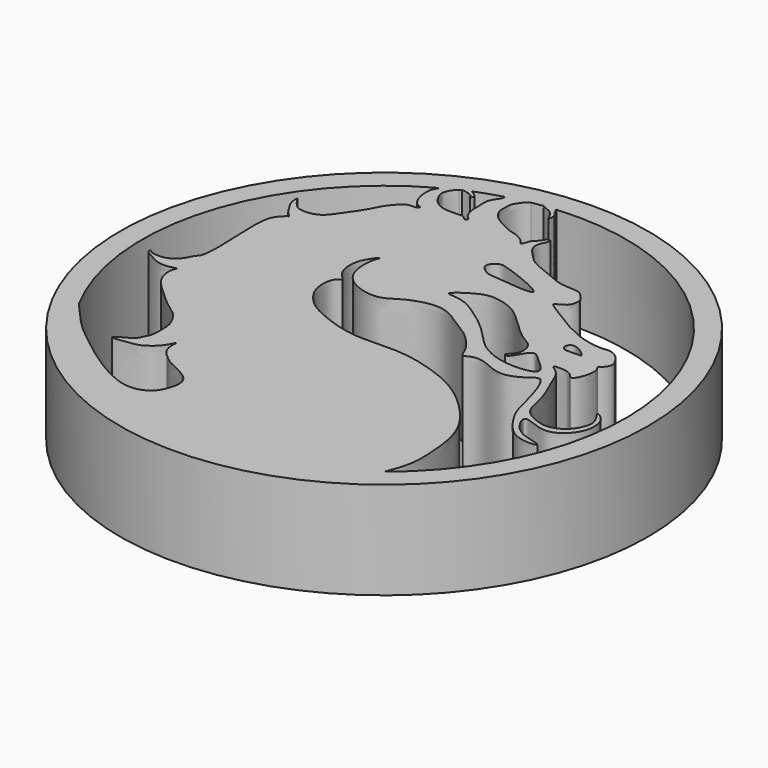
from build123d import *

# Parameters (mm, degrees)
F0_R     = 31.6990102439
F1_DEPTH = 11.7


with BuildPart() as f1:
    # F0 (on Top) → F1 (new body)
    with BuildSketch(Plane.XY):
        Circle(F0_R)
        with BuildLine():
            add(Edge.make_bspline(
                [(-25.4924991119, -13.953342914), (-24.5205169338, -15.0949653302), (-22.7712795464, -17.0908646211), (-20.9172889954, -18.6531879557), (-18.2968648266, -20.6691769997), (-16.0576388328, -22.2866539049), (-12.4835639639, -24.2367282269), (-10.1908173872, -24.1443080261), (-8.8516569375, -23.3219450661), (-8.2884059782, -22.1940801251), (-7.925939069, -20.9577066664), (-8.1157075896, -19.5625424569), (-9.9910246166, -18.4916373157), (-11.2641391672, -17.9900335901), (-12.2342182318, -17.2485160801), (-13.2039862501, -16.3164485705), (-13.4759813903, -15.2533092584), (-13.3229134314, -14.1868992615), (-13.7130330942, -15.0105365297), (-14.1891719411, -15.812497329), (-15.0326748195, -16.5008887465), (-15.8548336143, -17.0523376609), (-17.2619658719, -17.1641585773), (-17.9396597588, -17.310965029), (-19.0370830117, -17.4300508562), (-18.635512969, -16.9608620996), (-17.8651450299, -16.6343730103), (-17.1300961664, -16.1576111235), (-16.70189117, -15.7281851081), (-16.544862205, -15.1135475957), (-16.1178720626, -14.6375624469), (-16.1170114575, -12.1417295665), (-16.5073688058, -11.2488630843), (-17.1586601796, -10.0698478487), (-18.2395336648, -9.334157054), (-19.4351823142, -8.4220615411), (-20.9023358044, -7.0480236886), (-22.051850097, -6.0235129872), (-22.9560730456, -4.7224379727), (-23.1145722043, -3.1268944114), (-22.6189057646, -2.4703301229), (-23.4564204373, -2.768219693), (-24.2140705088, -2.8630415189), (-25.2546086687, -2.6946099421), (-26.1534811662, -2.0869842562), (-27.2257353007, -1.6017665898), (-27.0135812832, -1.1960557968), (-26.7692309783, -1.4218595095), (-26.6222190112, -1.5577130252)],
                knots=[0, 0, 0, 0, 0.0398660387, 0.0704586732, 0.1051574303, 0.1385907296, 0.1775557103, 0.2064699431, 0.2298732252, 0.2514273797, 0.2733952533, 0.2953631269, 0.3232816075, 0.3464860594, 0.3678132978, 0.3901099659, 0.4113282877, 0.427165272, 0.4411293294, 0.461100555, 0.4811676125, 0.5007036306, 0.5232544455, 0.5411884608, 0.5585369833, 0.5695176296, 0.5880729408, 0.6064731354, 0.6214715959, 0.6362150192, 0.6516876832, 0.6817388171, 0.7019175478, 0.7237519879, 0.7459225483, 0.7700142909, 0.7976991764, 0.8220278718, 0.8465425239, 0.8711245294, 0.8844079913, 0.8992487966, 0.9173023826, 0.9367348376, 0.95807413, 0.9778676473, 0.9866834549, 1, 1, 1, 1], degree=3))
            ThreePointArc((-25.4924991119, -13.953342914), (-27.8223142289, 8.2534102291), (-13.7385207838, 25.5801146426))
            add(Edge.make_bspline(
                [(-24.8989164829, -1.5577130252), (-24.6682612127, -1.4467950062), (-24.182278602, -1.2130946081), (-23.5284769239, -0.5252534093), (-23.1348921367, 0.5509903957), (-22.248480301, 0.9536932892), (-22.6348383075, 7.7223592702), (-22.6502976613, 8.636841393), (-22.5815628754, 10.3935904447), (-22.1575913528, 11.4418886666), (-21.3881202113, 12.1606956989), (-21.1235642698, 12.2680174337), (-21.8063168168, 12.7530703595), (-22.1396372934, 13.415098283), (-22.6935277447, 14.1650088888), (-22.8842543668, 14.8759577126), (-22.9465718409, 15.8082146545), (-22.559642771, 15.0793561333), (-22.1324554976, 14.5388286717), (-21.6979561921, 14.0895012776), (-20.9015910939, 13.8854920097), (-19.825223354, 13.9570235717), (-18.8458738409, 14.3881421588), (-18.071126134, 15.4033010207), (-17.2606622947, 16.5246614142), (-16.1601092221, 18.2494885912), (-15.6607329457, 19.3859623739), (-14.847256475, 20.4158034631), (-14.0235241732, 21.1839127113), (-12.9636520335, 21.0055073847), (-12.6225680971, 21.4021121154), (-13.3643600704, 21.5526818883), (-13.9976499307, 22.4695994422), (-14.3470936559, 24.0526739486), (-14.1182749531, 24.987729418), (-13.8062536012, 25.4899631194), (-13.7385207838, 25.5801146426)],
                knots=[0, 0, 0, 0, 0.0256023524, 0.0539148324, 0.0835052959, 0.1101156606, 0.1835979514, 0.2157474491, 0.2521308262, 0.2841448995, 0.3131193533, 0.3242716257, 0.3479291799, 0.3742971001, 0.4016912477, 0.4283317743, 0.4503249132, 0.4705478815, 0.4962303529, 0.5185566477, 0.5442746968, 0.5743387515, 0.603924567, 0.635986405, 0.6708293895, 0.7121609059, 0.7449046934, 0.77779553, 0.8080446572, 0.8370290557, 0.8523168513, 0.8735942078, 0.9042708295, 0.9410102592, 0.9713895558, 0.988723741, 0.988723741, 0.988723741, 0.988723741], degree=3))
            ThreePointArc((-24.8989164829, -1.5577130252), (-25.7605677471, -1.6476774835), (-26.6222190112, -1.5577130252))
        make_face(mode=Mode.SUBTRACT)
        with BuildLine():
            add(Edge.make_bspline(
                [(-10.9293263316, 26.9279244537), (-10.7761460856, 27.1829858205), (-8.4632358732, 28.0968939132), (-7.96494233, 27.9485774795)],
                knots=[0.9212322924, 0.9212322924, 0.9212322924, 0.9212322924, 1, 1, 1, 1], degree=3))
            add(Edge.make_bspline(
                [(-7.96494233, 27.9485774795), (-7.7659081919, 27.8893352237), (-7.9854693758, 27.334327223), (-8.6107966287, 26.6199241698), (-8.6776661013, 25.6673183501), (-8.6392304428, 24.6062468981), (-8.6222883478, 23.8891934323), (-8.3826328059, 23.0456884712), (-8.0681070278, 22.5984307712), (-7.6157977084, 22.3314622086), (-7.9749634219, 21.8869519667), (-8.4100164684, 22.5647023154), (-8.9115097447, 22.4367696203), (-10.1307278197, 22.4487455576), (-11.0349709889, 22.4817336074), (-12.0373032391, 23.0359552222), (-12.6025375261, 23.7829307418), (-13.085013525, 24.7626616584), (-12.7917248315, 25.607226175), (-12.3580057447, 26.2480317748), (-12.1076796932, 26.4115543799)],
                knots=[0, 0, 0, 0, 0.0314623037, 0.0763474099, 0.1193264625, 0.1649299311, 0.2031829971, 0.2440939774, 0.2776170473, 0.306375695, 0.3307447355, 0.3653371172, 0.3961799588, 0.4448777919, 0.4881595176, 0.5342293817, 0.5777229306, 0.6224266783, 0.6654307938, 0.7043560235, 0.7043560235, 0.7043560235, 0.7043560235], degree=3))
            add(Edge.make_bspline(
                [(-12.1076796932, 26.4115543799), (-12.0517851626, 26.4480668372), (-11.9623289371, 26.4934654527), (-11.8679265331, 26.5179265415), (-11.8343802261, 26.5242422913)],
                knots=[0.7043560235, 0.7043560235, 0.7043560235, 0.7043560235, 0.7130475178, 0.7177379547, 0.7177379547, 0.7177379547, 0.7177379547], degree=3))
            add(Edge.make_bspline(
                [(-11.8343802261, 26.5242422913), (-11.559754757, 26.5759459183), (-10.9875568221, 26.3892344151), (-10.4576202112, 26.2366404817), (-10.3900777933, 25.6244407913), (-10.0684688917, 26.2862308156), (-10.4630411207, 26.5381919596), (-10.741933352, 26.8073503852), (-10.9661388399, 26.8666277204), (-10.9293263316, 26.9279244537)],
                knots=[0.7177379547, 0.7177379547, 0.7177379547, 0.7177379547, 0.7561360243, 0.7897031721, 0.8152486256, 0.8441184845, 0.8729606375, 0.9023027178, 0.9212322924, 0.9212322924, 0.9212322924, 0.9212322924], degree=3))
        make_face(mode=Mode.SUBTRACT)
        with BuildLine():
            add(Edge.make_bspline(
                [(-2.484705373, 28.9549568927), (-2.4451644444, 28.8651249424), (-2.3596546867, 28.6588472844), (-2.1613804441, 28.2044873265), (-1.9646475399, 28.107947855), (-1.7867933838, 27.8151547157), (-1.8415957155, 26.7655274123), (-2.1794564322, 27.6203453266), (-2.6094919673, 28.1945682393), (-3.0558420117, 28.4400351672), (-3.5441074181, 28.5924201729), (-3.7220759765, 28.7622909996), (-3.8972114787, 28.7988720636)],
                knots=[0, 0, 0, 0, 0.0104528451, 0.0230253936, 0.0310733894, 0.0420287589, 0.0570681944, 0.0702000837, 0.0864992161, 0.0993078833, 0.1118944012, 0.1237250051, 0.1237250051, 0.1237250051, 0.1237250051], degree=3))
            ThreePointArc((-2.484705373, 28.9549568927), (27.0029867302, 10.7425321546), (18.0845215617, -22.7489201795))
            add(Edge.make_bspline(
                [(21.0905393961, 8.2323806828), (21.2092121617, 8.0450376225), (21.4793193775, 7.6196538743), (20.8753393499, 6.5979428882), (20.3647799435, 6.5195460728), (20.8289691335, 5.9894389958), (20.9002170042, 5.1521028751), (20.5463161677, 3.741749083), (19.886314193, 2.9495578524), (19.4490916193, 3.6933796284), (18.6554250994, 4.0537538147), (17.7853422575, 4.0391452824), (16.8750029658, 4.0311784039), (18.0475158101, 3.3271116272), (18.6818393044, 2.3800689137), (19.3312582634, 0.7195463097), (20.0303141079, -0.8442092267), (20.5571848976, -2.5555691151), (20.8696843515, -4.5706503487), (22.3292649832, -5.4996025705), (23.90557084, -6.0612209947), (25.2863092919, -5.8100773386), (26.5363535881, -4.9849813224), (27.2580149423, -3.4956580916), (27.3441321447, -2.26276688), (26.0258920594, -0.6584704762), (27.4528740596, -1.4974288954), (27.9100462677, -2.9011266287), (27.7006899586, -4.6560332158), (26.4299516449, -6.2226163533), (24.4108929347, -7.144583982), (21.1064401244, -5.2565510426), (22.2721522236, -7.8605103151), (23.8851547148, -8.8785208204), (25.6078181678, -9.1573838999), (26.2064164148, -9.5825351957), (24.4112882164, -9.6937583109), (22.763138848, -9.0875288524), (21.4318436368, -7.5853237787), (20.1421912098, -5.5535853082), (19.616326949, -3.2406831016), (19.0069108519, -0.9587342144), (17.9023835586, 1.7117840189), (16.6577260619, 0.4883223848), (14.1753194999, -0.723546406), (11.9111345021, 0.6195556277), (10.1428376279, 0.9095226228), (9.0327799793, 0.0440375637), (8.7801335009, 1.4957269354), (6.8664962017, 3.7536041529), (4.8926069045, 4.8894613094), (2.3533656526, 6.6795065111), (0.0001395771, 6.7148314368), (-2.4704605059, 5.8050123315), (-4.0610881428, 4.5164236847), (-6.3303899278, 4.6501809763), (-8.4841075846, 5.6411819065), (-9.6734661214, 7.540250021), (-9.6357379143, 10.1321245172), (-8.9927696704, 11.3862113102), (-10.183758132, 9.9755575402), (-10.7383454542, 8.2936077105), (-10.3097754053, 6.1896125354), (-9.03755311, 5.3583600586), (-10.1668804683, 4.8911710786), (-10.2814373087, 2.4760959142), (-9.147351654, 0.6187240927), (-7.3825594604, -1.0061326079), (-3.3539419066, -2.4854568434), (-0.473332675, -2.9410325472), (4.1739938603, -2.5544606803), (8.3297649823, -3.5876850226), (12.196826759, -5.0851354647), (16.0677267209, -8.4047507302), (18.7811144093, -12.226083744), (19.2321354076, -17.4563600104), (19.1671718864, -20.2402936026), (18.2007436749, -22.5931512702), (18.0845215617, -22.7489201795)],
                knots=[0, 0, 0, 0, 0.0079496706, 0.0180530351, 0.0237091293, 0.0305562386, 0.0396071702, 0.0516221641, 0.0600139438, 0.0677222737, 0.0767801533, 0.0863654962, 0.0932811022, 0.1025550398, 0.1135184432, 0.126388158, 0.1392077086, 0.1523367497, 0.1658744702, 0.1782839748, 0.1907586248, 0.2020294739, 0.213752193, 0.2259660295, 0.2371754568, 0.2483165269, 0.2573472845, 0.2694534839, 0.282109495, 0.2955635266, 0.3100238289, 0.3255757422, 0.3378386484, 0.3521020436, 0.364951246, 0.370468792, 0.3816878817, 0.3950514604, 0.408633495, 0.4236841109, 0.4385315646, 0.4542685642, 0.4688622342, 0.4795260512, 0.4953270069, 0.510791214, 0.5236724239, 0.5332040151, 0.5430786338, 0.5597970581, 0.5749607294, 0.5917227346, 0.6064536898, 0.6220611062, 0.6357591425, 0.6499525087, 0.6646862325, 0.6789842566, 0.6949297022, 0.7032332358, 0.7137384412, 0.7274080051, 0.7414764617, 0.7515301697, 0.759908862, 0.7743646549, 0.7886402458, 0.8036378116, 0.8234941102, 0.8404411389, 0.8611598626, 0.8813585256, 0.9010797519, 0.9228402178, 0.9439405737, 0.9657232287, 0.9830511585, 0.9979085503, 0.9979085503, 0.9979085503, 0.9979085503], degree=3))
            add(Edge.make_bspline(
                [(-5.2045053557, 28.5915444397), (-5.5758718219, 28.4160946747), (-6.0053962059, 27.9023065803), (-6.4897099552, 27.0973386243), (-6.4970616336, 26.4878198164), (-6.5457985627, 25.5616410141), (-6.2886066932, 25.0188944529), (-6.0105651908, 24.5301914717), (-5.3997621058, 23.9935066472), (-4.7098020912, 23.591285149), (-3.9482439749, 23.2459970906), (-3.352217994, 22.8660204582), (-2.464211201, 22.7428046132), (-1.7055443941, 22.3551921416), (-1.1017385976, 21.989631285), (-0.7070662853, 21.2226665424), (-0.4766619461, 22.2784381642), (-0.1904600163, 22.6895292306), (0.3080197232, 23.0613227622), (0.5779244584, 23.8035283207), (0.9922780128, 23.695981916), (1.0384229302, 23.7355183291), (0.9960349297, 23.1397299358), (0.694611579, 22.7497285866), (0.4781450599, 21.975078267), (0.7111891962, 21.3867857223), (0.935205971, 20.9923488328), (1.4161405679, 20.5382887259), (2.3451134665, 19.4459822716), (3.6221697585, 18.8518898044), (5.3018841384, 18.2045655961), (7.212414579, 17.2698647622), (9.4075652816, 17.3880331414), (10.0219686643, 16.9502229586), (10.8563855381, 15.9838347802), (10.7841877573, 15.4188711339), (10.6323129048, 14.5787876054), (9.9531215816, 14.2756240504), (9.6228271691, 13.998293694), (8.9377839878, 13.8136054102), (10.9189488754, 12.667341263), (12.4354181486, 11.7058759376), (13.0933969472, 11.2651494217), (13.7445850808, 10.9444229563), (14.4147315421, 10.724919445), (15.1836717831, 10.2434398899), (16.1792986059, 9.9640718543), (16.8489198791, 9.790311513), (17.8124414535, 9.6530132891), (18.5526372647, 9.6085049239), (19.1125094729, 9.7256381992), (19.7504845974, 9.6369581864), (20.3688544295, 9.2288185047), (20.8005719924, 8.8239106123), (21.0952490672, 8.2680338686), (21.0912269507, 8.2348932271), (21.0905393961, 8.2323806828)],
                knots=[0.1446417047, 0.1446417047, 0.1446417047, 0.1446417047, 0.1635828728, 0.1806641402, 0.1948959541, 0.2121766804, 0.2261299557, 0.2395781086, 0.2557995351, 0.2722508569, 0.288758187, 0.3039771815, 0.3209966621, 0.3377560807, 0.3536386939, 0.3666034692, 0.3822757442, 0.3959144594, 0.4101462549, 0.4254823851, 0.4356687402, 0.4381371501, 0.4507653719, 0.4644802678, 0.480285874, 0.4945176604, 0.5064388429, 0.521013825, 0.542548481, 0.5641771572, 0.5884266857, 0.6154320691, 0.6414918635, 0.6572351016, 0.676916846, 0.6905086183, 0.7066095356, 0.7216935533, 0.7342002987, 0.7447284474, 0.7692803231, 0.7952140281, 0.8109689845, 0.8260899649, 0.8413020202, 0.8586839438, 0.8770233214, 0.8923437088, 0.9101833494, 0.9258887987, 0.9394349169, 0.9537847552, 0.9691592912, 0.9840690543, 0.9977969664, 0.99930344, 0.99930344, 0.99930344, 0.99930344], degree=3))
            add(Edge.make_bspline(
                [(-3.8972114787, 28.7988720636), (-4.2068538878, 28.8635479782), (-4.794406, 28.7852933162), (-5.2045053557, 28.5915444397)],
                knots=[0.1237250051, 0.1237250051, 0.1237250051, 0.1237250051, 0.1446417047, 0.1446417047, 0.1446417047, 0.1446417047], degree=3))
        make_face(mode=Mode.SUBTRACT)
        with BuildLine():
            add(Edge.make_bspline(
                [(16.7020484805, 2.4024655577), (16.7034081895, 2.1889414303), (16.2155004354, 1.7506183906), (14.1861074704, 1.5551250062), (11.9607993516, 1.8845696747), (9.4890471208, 2.990010419), (7.2680237364, 5.6967240949), (4.8638926969, 7.5318814462), (2.4921442293, 9.0979298015), (0.8781997115, 9.2479125231), (-0.2365899848, 9.318228571), (2.5899771203, 11.3243581389), (4.3837213326, 11.4614775235), (6.8865893852, 10.7677530326), (8.9935753573, 8.8046685713), (11.2277146443, 6.6092285294), (12.9093651761, 6.0041564801), (13.1709998773, 3.8459879705), (11.8226771988, 3.0258316055), (12.7667544841, 2.6454011652), (13.7239460337, 5.4753960646), (15.000385052, 4.3285889657), (16.0178340348, 3.4881170264), (16.7002467424, 2.6854044483), (16.7020484805, 2.4024655577)],
                knots=[0, 0, 0, 0, 0.0273165284, 0.0743590864, 0.1249451523, 0.1790159508, 0.2410433094, 0.300018134, 0.3558570466, 0.3988075372, 0.4219052761, 0.4765519636, 0.5241691681, 0.575690919, 0.6331373107, 0.6920252162, 0.7349081981, 0.779946638, 0.8155179704, 0.8362574318, 0.8874773816, 0.9225440156, 0.9638031152, 1, 1, 1, 1], degree=3))
        make_face(mode=Mode.SUBTRACT)
        with BuildLine():
            add(Edge.make_bspline(
                [(6.2505416572, 14.5358983427), (6.428305526, 14.956919891), (1.3429650228, 16.9838826529), (0.05938938, 17.133201532), (-0.8415581091, 15.918420386), (-0.0127338665, 15.1686838172), (0.6362383264, 14.7435926409), (1.2630715432, 14.7238080855), (6.0796460576, 14.1311438196), (6.2505416572, 14.5358983427)],
                knots=[0, 0, 0, 0, 0.2398079028, 0.3718784462, 0.4804859486, 0.5828934206, 0.6701043834, 0.7694575641, 1, 1, 1, 1], degree=3))
        make_face(mode=Mode.SUBTRACT)
        with BuildLine():
            add(Edge.make_bspline(
                [(17.837703228, 7.3236334138), (17.8120348188, 7.5314910144), (16.2735075614, 8.7560982134), (15.3706837141, 8.0865343977), (15.628484938, 7.0279072071), (17.199175351, 7.317048782), (17.8514026615, 7.2126981642), (17.837703228, 7.3236334138)],
                knots=[0, 0, 0, 0, 0.2679330895, 0.4477435398, 0.6133768728, 0.8570019858, 1, 1, 1, 1], degree=3))
        make_face(mode=Mode.SUBTRACT)
        with BuildLine():
            ThreePointArc((-10.9293263316, 26.9279244537), (-9.4609080016, 27.4782552072), (-7.96494233, 27.9485774795))
            add(Edge.make_bspline(
                [(-10.9293263316, 26.9279244537), (-10.7761460856, 27.1829858205), (-8.4632358732, 28.0968939132), (-7.96494233, 27.9485774795)],
                knots=[0.9212322924, 0.9212322924, 0.9212322924, 0.9212322924, 1, 1, 1, 1], degree=3))
        make_face()
        with BuildLine():
            add(Edge.make_bspline(
                [(-12.1076796932, 26.4115543799), (-12.0517851626, 26.4480668372), (-11.9623289371, 26.4934654527), (-11.8679265331, 26.5179265415), (-11.8343802261, 26.5242422913)],
                knots=[0.7043560235, 0.7043560235, 0.7043560235, 0.7043560235, 0.7130475178, 0.7177379547, 0.7177379547, 0.7177379547, 0.7177379547], degree=3))
            Line((-12.1076796932, 26.4115543799), (-11.8343802261, 26.5242422913))
        make_face()
        with BuildLine():
            ThreePointArc((-5.2045053557, 28.5915444397), (-4.5520389409, 28.7026519842), (-3.8972114787, 28.7988720636))
            add(Edge.make_bspline(
                [(-3.8972114787, 28.7988720636), (-4.2068538878, 28.8635479782), (-4.794406, 28.7852933162), (-5.2045053557, 28.5915444397)],
                knots=[0.1237250051, 0.1237250051, 0.1237250051, 0.1237250051, 0.1446417047, 0.1446417047, 0.1446417047, 0.1446417047], degree=3))
        make_face()
    extrude(amount=F1_DEPTH)


solid = f1.part
